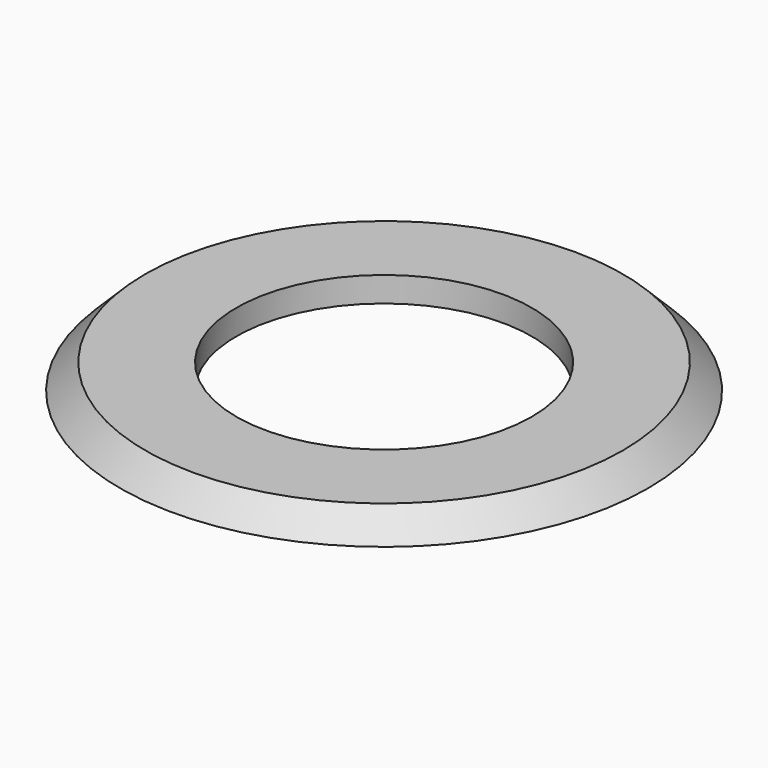
from build123d import *

# Parameters (mm, degrees)
F0_R     = 10.5
F0_R_2   = 5.875
F1_DEPTH = 1
F2_SIZE  = 0.99999


# Not quite as in the source:
# - a fillet or chamfer is up to 0.001 mm smaller than in the source, because OpenCascade refuses the exact size


with BuildPart() as f1:
    # F0 (on Top) → F1 (new body)
    with BuildSketch(Plane.XY):
        Circle(F0_R)
        Circle(F0_R_2, mode=Mode.SUBTRACT)
    extrude(amount=F1_DEPTH)

    # F2 (size 1 in the source; OpenCascade refuses exactly that, so slightly less here)
    f2_edges = [f1.edges().sort_by_distance(p)[0] for p in [
        (-10.5, 0, 1),
    ]]
    chamfer(f2_edges, length=F2_SIZE)


solid = f1.part
